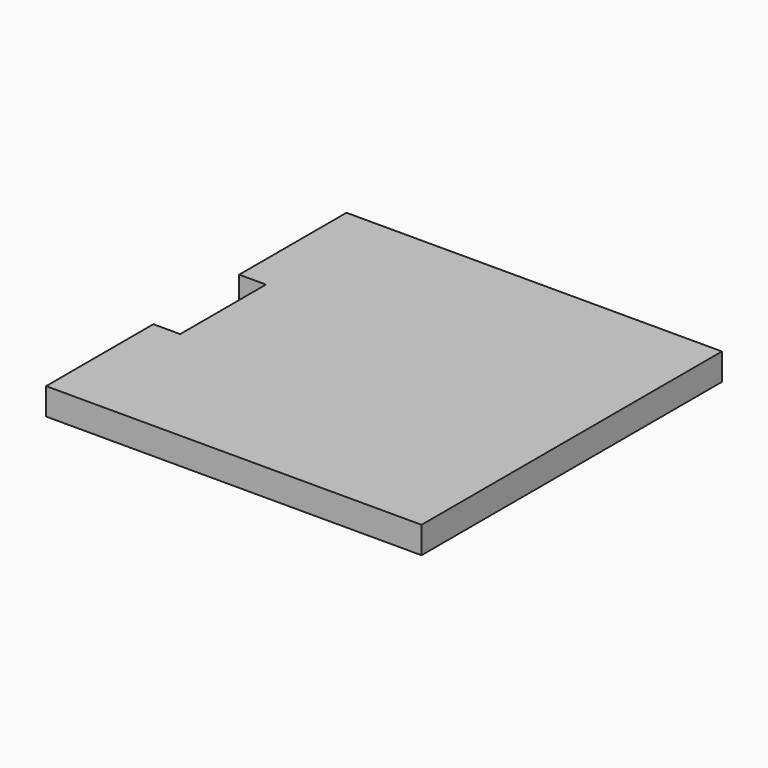
from build123d import *

# Parameters (mm, degrees)
F1_DEPTH = 1.5875


# Not quite as in the source:
# - a length typed as a fraction of an inch, garbled in the dataset ("3 / 203.2 mm" for 3/8 in), is restored


with BuildPart() as f1:
    # F0 (on Top) → F1 (new body)
    with BuildSketch(Plane.XY):
        Polygon((-11.1125, -3.175), (-11.1125, -11.1125), (11.1125, -11.1125), (11.1125, 11.1125), (-11.1125, 11.1125), (-11.1125, 3.175), (-9.525, 3.175), (-9.525, -3.175), align=None)
    extrude(amount=F1_DEPTH)


solid = f1.part
